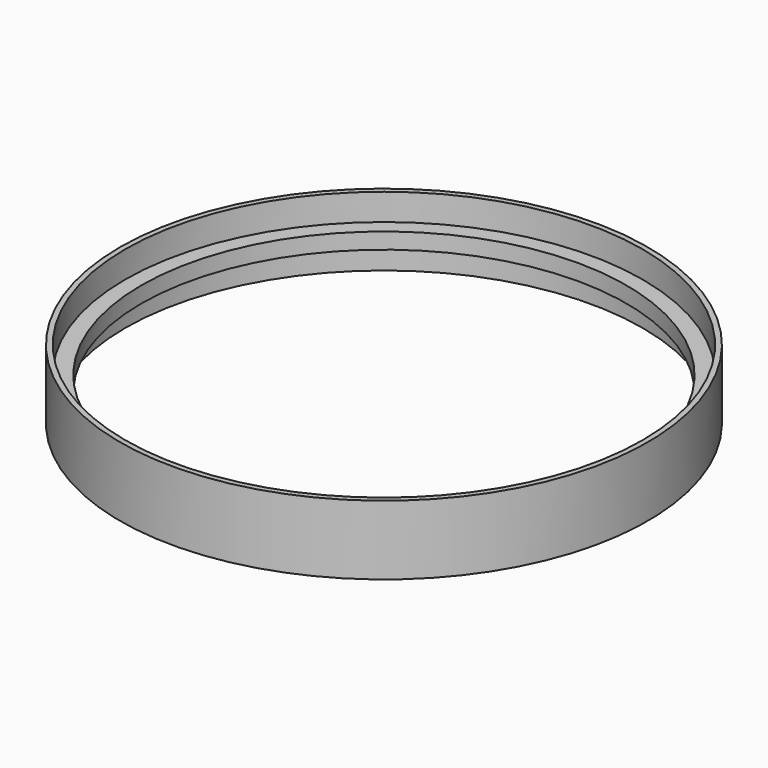
from build123d import *

# Parameters (mm, degrees)
F2_R     = 1
F3_DEPTH = 48.006


# Not quite as in the source:
# - the program builds the solid bodies; features that only make, move or delete a surface that nothing else refers to are left out


with BuildPart() as f1:
    # F0 (on Front) → F1 (revolve)
    with BuildSketch(Plane.XZ):
        Polygon((-48.5, 6.5), (-49.5, 6.5), (-49.5, -6.5), (-48.5, -6.5), (-48.5, -1.5), (-45.5, -1.5), (-45.5, 0), (-45.5, 1.5), (-48.5, 1.5), align=None)
    revolve(axis=Axis((0, 0, -3.8321989188), (0, 0, -1)))

    # F2 (on Right) → F3 (cut)
    with BuildSketch(Plane.YZ):
        with Locations((-3, 0)):
            Circle(F2_R)
        with BuildLine():
            ThreePointArc((4, 0), (3, 1), (2, 0))
            ThreePointArc((2, 0), (3, -1), (4, 0))
        make_face()
    extrude(amount=F3_DEPTH, mode=Mode.SUBTRACT)


solid = f1.part
